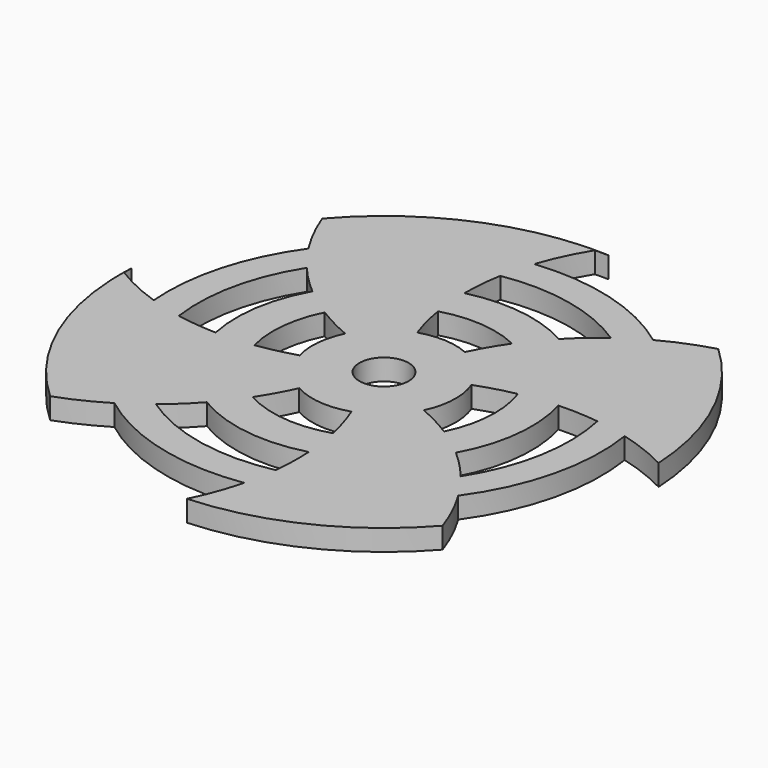
from build123d import *

# Parameters (mm, degrees)
F0_R     = 3.5
F1_DEPTH = 3


# Not quite as in the source:
# - a feature names something its author has since deleted; it is built from what else it names


with BuildPart() as f1:
    # F0 (on Top) → F1 (new body)
    with BuildSketch(Plane.XY):
        with BuildLine():
            Line((-103.8872403759, 50.9688953831), (-101.9313409925, 50.9688953831))
            Line((-101.9313409925, 50.9688953831), (-99.975441609, 50.9688953831))
            ThreePointArc((-99.975441609, 50.9688953831), (-101.9313409925, 51.0198679723), (-103.8872403759, 50.9688953831))
        make_face()
        with BuildLine():
            ThreePointArc((-105.128088395, 44.1726214205), (-103.7275117352, 47.6637957311), (-101.9313409925, 50.9688953831))
            Line((-101.9313409925, 50.9688953831), (-103.8872403759, 50.9688953831))
            ThreePointArc((-103.8872403759, 50.9688953831), (-118.4470490216, 47.1928769199), (-130.3569155648, 38.005852257))
            ThreePointArc((-130.3569155648, 38.005852257), (-128.876069776, 34.6235055457), (-127.0483694881, 31.4152840472))
            ThreePointArc((-127.0483694881, 31.4152840472), (-131.6855143995, 21.6924682926), (-132.6995872702, 10.9682939496))
            ThreePointArc((-132.6995872702, 10.9682939496), (-136.152020588, 12.3518590173), (-139.4313409925, 14.1067395817))
            Line((-139.4313409925, 14.1067395817), (-139.4313409925, 11.5129959997))
            ThreePointArc((-139.4313409925, 11.5129959997), (-135.8835245013, -2.5724504886), (-127.2555101816, -14.2576622337))
            ThreePointArc((-127.2555101816, -14.2576622337), (-123.8698155437, -12.8388675837), (-120.6478658456, -11.079621557))
            ThreePointArc((-120.6478658456, -11.079621557), (-109.6296820224, -16.4254775309), (-97.3998915176, -17.0663948921))
            ThreePointArc((-97.3998915176, -17.0663948921), (-98.4971319541, -20.6192094649), (-99.975441609, -24.0311046169))
            ThreePointArc((-99.975441609, -24.0311046169), (-85.5790985856, -20.3346504467), (-73.7446837693, -11.342148468))
            ThreePointArc((-73.7446837693, -11.342148468), (-75.1429207557, -7.8890051383), (-76.9083449574, -4.6083736574))
            ThreePointArc((-76.9083449574, -4.6083736574), (-71.9248057865, 6.2200450283), (-71.4154696243, 18.1293225284))
            ThreePointArc((-71.4154696243, 18.1293225284), (-67.8499010769, 16.9668747828), (-64.4313409925, 15.4247947665))
            ThreePointArc((-64.4313409925, 15.4247947665), (-67.9189218222, 29.3821252434), (-76.3988312093, 41.0037185452))
            ThreePointArc((-76.3988312093, 41.0037185452), (-79.9768515125, 39.773669955), (-83.3966724505, 38.1550058214))
            ThreePointArc((-83.3966724505, 38.1550058214), (-93.6932659385, 43.219056827), (-105.128088395, 44.1726214205))
        make_face()
        with BuildLine():
            ThreePointArc((-116.8786483854, -8.4112257418), (-114.7452282061, -6.5377141597), (-112.7675725108, -4.500459816))
            ThreePointArc((-112.7675725108, -4.500459816), (-104.8400955118, -7.312365092), (-96.445234408, -6.785098651))
            ThreePointArc((-96.445234408, -6.785098651), (-96.3945126034, -9.6374635235), (-96.5828731928, -12.4840541783))
            ThreePointArc((-96.5828731928, -12.4840541783), (-107.144920689, -12.5114873217), (-116.8786483854, -8.4112257418))
        make_face(mode=Mode.SUBTRACT)
        with BuildLine():
            ThreePointArc((-97.1633932868, -1.5770140117), (-103.489663028, -2.237292801), (-109.5628503108, -0.3467761664))
            ThreePointArc((-109.5628503108, -0.3467761664), (-108.1146014235, 2.0457215346), (-106.8582364184, 4.544324557))
            ThreePointArc((-106.8582364184, 4.544324557), (-102.9079011749, 3.321551239), (-98.7968737544, 3.768515076))
            ThreePointArc((-98.7968737544, 3.768515076), (-97.870198127, 1.1293444599), (-97.1633932868, -1.5770140117))
        make_face(mode=Mode.SUBTRACT)
        with BuildLine():
            ThreePointArc((-87.020290304, 18.643185886), (-86.1794714129, 12.4732450474), (-87.7904785909, 6.4582801904))
            ThreePointArc((-87.7904785909, 6.4582801904), (-90.2129680661, 7.8584356684), (-92.7417733998, 9.0559473403))
            ThreePointArc((-92.7417733998, 9.0559473403), (-91.7456646982, 13.0514491022), (-92.4114813686, 17.1150626462))
            ThreePointArc((-92.4114813686, 17.1150626462), (-89.7469190596, 17.9886089148), (-87.020290304, 18.643185886))
        make_face(mode=Mode.SUBTRACT)
        with BuildLine():
            ThreePointArc((-79.6045613776, -0.8026360965), (-81.5030217359, 1.3342277264), (-83.5732367524, 3.3051535278))
            ThreePointArc((-83.5732367524, 3.3051535278), (-81.0808826805, 11.1066871006), (-81.7647527708, 19.2680642275))
            ThreePointArc((-81.7647527708, 19.2680642275), (-78.8888619154, 19.2681720991), (-76.0229262651, 19.0290882807))
            ThreePointArc((-76.0229262651, 19.0290882807), (-75.8548608571, 8.7594492912), (-79.6045613776, -0.8026360965))
        make_face(mode=Mode.SUBTRACT)
        with BuildLine():
            ThreePointArc((-124.2925325258, 27.6864483354), (-122.366283457, 25.5897237243), (-120.2765526126, 23.655889562))
            ThreePointArc((-120.2765526126, 23.655889562), (-122.6767843834, 16.6229750116), (-122.4752234892, 9.1944911263))
            ThreePointArc((-122.4752234892, 9.1944911263), (-125.3358583127, 9.3662040749), (-128.1716299117, 9.7798662184))
            ThreePointArc((-128.1716299117, 9.7798662184), (-127.8289740179, 19.0790916737), (-124.2925325258, 27.6864483354))
        make_face(mode=Mode.SUBTRACT)
        with BuildLine():
            ThreePointArc((-116.0346336158, 20.5547864365), (-113.602585651, 19.1733015065), (-111.068333377, 17.9896954377))
            ThreePointArc((-111.068333377, 17.9896954377), (-112.0801205218, 14.4304238708), (-111.7547699117, 10.7444675099))
            ThreePointArc((-111.7547699117, 10.7444675099), (-114.4574555109, 10.0161737122), (-117.2111759917, 9.514232662))
            ThreePointArc((-117.2111759917, 9.514232662), (-117.6257828154, 15.1413817681), (-116.0346336158, 20.5547864365))
        make_face(mode=Mode.SUBTRACT)
        with Locations((-101.9313409925, 13.4688953831)):
            Circle(F0_R, mode=Mode.SUBTRACT)
        with BuildLine():
            ThreePointArc((-106.3733358176, 28.6142377963), (-100.6487081208, 29.1999973076), (-95.0945804167, 27.6946262842))
            ThreePointArc((-95.0945804167, 27.6946262842), (-96.6062830352, 25.3254140346), (-97.9178620412, 22.8398211472))
            ThreePointArc((-97.9178620412, 22.8398211472), (-101.4213565394, 23.6503578923), (-104.988310348, 23.1939764279))
            ThreePointArc((-104.988310348, 23.1939764279), (-105.7981495503, 25.8741269811), (-106.3733358176, 28.6142377963))
        make_face(mode=Mode.SUBTRACT)
        with BuildLine():
            ThreePointArc((-87.3838790757, 35.6168761154), (-89.634828263, 33.8018778137), (-91.7240079261, 31.8027981717))
            ThreePointArc((-91.7240079261, 31.8027981717), (-99.0699795968, 34.2567343942), (-106.8057550879, 33.8787392584))
            ThreePointArc((-106.8057550879, 33.8787392584), (-106.6786212529, 36.7532837824), (-106.296701705, 39.6051790629))
            ThreePointArc((-106.296701705, 39.6051790629), (-96.4636690625, 39.3969933158), (-87.3838790757, 35.6168761154))
        make_face(mode=Mode.SUBTRACT)
        with BuildLine():
            Line((-139.4313409925, 14.1067395817), (-139.4313409925, 15.4247947665))
            ThreePointArc((-139.4313409925, 15.4247947665), (-139.4594284478, 14.7796945074), (-139.4764192758, 14.1342066599))
            ThreePointArc((-139.4764192758, 14.1342066599), (-139.4538855016, 14.1204643119), (-139.4313409925, 14.1067395817))
        make_face()
        with BuildLine():
            Line((-139.4313409925, 11.5129959997), (-139.4313409925, 14.1067395817))
            ThreePointArc((-139.4313409925, 14.1067395817), (-139.4538855016, 14.1204643119), (-139.4764192758, 14.1342066599))
            ThreePointArc((-139.4764192758, 14.1342066599), (-139.4767618846, 12.8232078208), (-139.4313409925, 11.5129959997))
        make_face()
    extrude(amount=F1_DEPTH)


solid = f1.part
